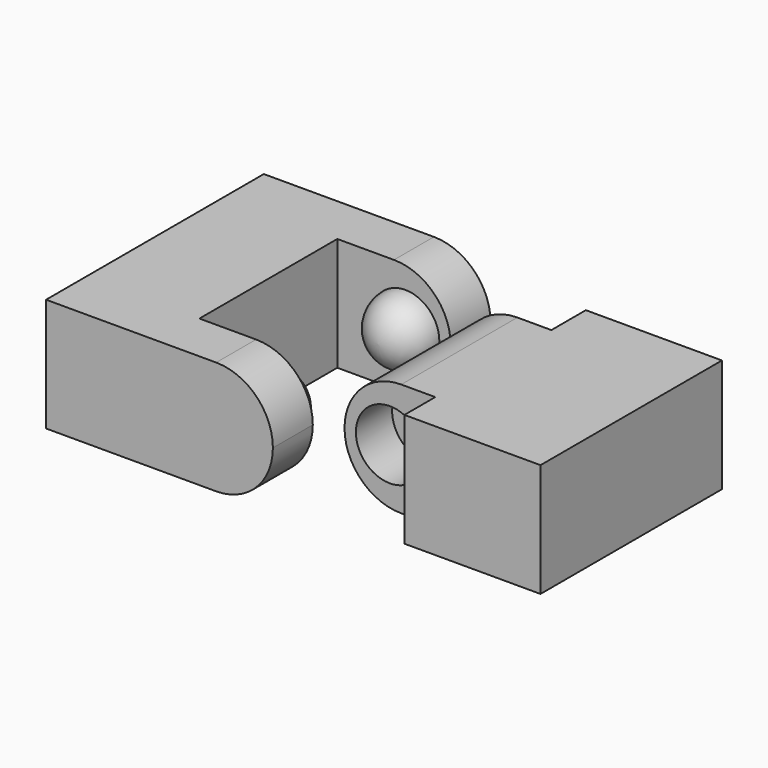
from build123d import *

# Parameters (mm, degrees)
F1_DEPTH  = 5
F2_R      = 1.5
F3_DEPTH  = 1.5
F4_R      = 1.5
F5_DEPTH  = 2
F6_R      = 1.5
F7_DEPTH  = 1.5
F8_R      = 1.49999
F9_W      = 1
F9_H      = 7.6
F10_DEPTH = 5
F11_DEPTH = 1
F12_DEPTH = 1
F13_R     = 2.49999
F13_2_R   = 2.49999
F14_DEPTH = 2
F15_DEPTH = 2
F16_R     = 1.5
F17_DEPTH = 2


# Not quite as in the source:
# - a fillet or chamfer is up to 0.001 mm smaller than in the source, because OpenCascade refuses the exact size


with BuildPart() as f1:
    # F0 (on Top) → F1 (new body)
    with BuildSketch(Plane.XY):
        Polygon((0, 6.4), (0, 0), (4, 0), (4, -1.7), (8, -1.7), (8, 8.3), (4, 8.3), (4, 6.4), align=None)
    extrude(amount=F1_DEPTH)

    # F4 (on face) → F5 (cut)
    with BuildSketch(Plane(origin=(0, 6.4, 0), x_dir=(-1, 0, 0), z_dir=(0, 1, 0))):
        with Locations((-2, 2.5)):
            Circle(F4_R)
    extrude(amount=-F5_DEPTH, mode=Mode.SUBTRACT)

    # F13 (radius 2.5 in the source; OpenCascade refuses exactly that, so slightly less here)
    f13_edges = [f1.edges().sort_by_distance(p)[0] for p in [
        (0, 3.2, 5),
        (0, 3.2, 0),
    ]]
    fillet(f13_edges, radius=F13_R)

    # F14 (add): a face of the model
    f14_faces = [f1.faces().sort_by_distance(p)[0] for p in [
        (8, 3.3, 2.5),
    ]]
    extrude(f14_faces, amount=F14_DEPTH)

    # F16 (on face) → F17 (cut)
    with BuildSketch(Plane.XZ):
        with Locations((2, 2.5)):
            Circle(F16_R)
    extrude(amount=-F17_DEPTH, mode=Mode.SUBTRACT)


with BuildPart() as f1b:
    # F0 (on Top) → F1, piece 2 (new body)
    with BuildSketch(Plane.XY):
        Polygon((-5, 7.1), (-1, 7.1), (-1, 8.3), (-9, 8.3), (-9, -1.7), (-1, -1.7), (-1, -0.5), (-5, -0.5), align=None)
    extrude(amount=F1_DEPTH)

    # F2 (on face) → F3 (join)
    with BuildSketch(Plane.XZ.offset(-7.1)):
        with Locations((-3, 2.5)):
            Circle(F2_R)
    extrude(amount=F3_DEPTH)

    # F6 (on face) → F7 (join)
    with BuildSketch(Plane(origin=(0, -0.5, 0), x_dir=(-1, 0, 0), z_dir=(0, 1, 0))):
        with Locations((3, 2.5)):
            Circle(F6_R)
    extrude(amount=F7_DEPTH)

    # F8 (radius 1.5 in the source; OpenCascade refuses exactly that, so slightly less here)
    f8_edges = [f1b.edges().sort_by_distance(p)[0] for p in [
        (-1.5, 1, 2.5),
        (-4.5, 5.6, 2.5),
    ]]
    fillet(f8_edges, radius=F8_R)

    # F9 (on face) → F10 (cut, through all)
    with BuildSketch(Plane.XY.offset(5)):
        with Locations((-5.5, 3.3)):
            Rectangle(F9_W, F9_H)
    extrude(amount=-F10_DEPTH, mode=Mode.SUBTRACT)

    # F11 (add): a face of the model
    f11_faces = [f1b.faces().sort_by_distance(p)[0] for p in [
        (-5, -1.7, 2.5),
    ]]
    extrude(f11_faces, amount=F11_DEPTH)

    # F12 (add): a face of the model
    f12_faces = [f1b.faces().sort_by_distance(p)[0] for p in [
        (-5, 8.3, 2.5),
    ]]
    extrude(f12_faces, amount=F12_DEPTH)

    # F13#2 (radius 2.5 in the source; OpenCascade refuses exactly that, so slightly less here)
    f13_2_edges = [f1b.edges().sort_by_distance(p)[0] for p in [
        (-1, -1.6, 0),
        (-1, -1.6, 5),
        (-1, 8.2, 5),
        (-1, 8.2, 0),
    ]]
    fillet(f13_2_edges, radius=F13_2_R)

    # F15 (add): a face of the model
    f15_faces = [f1b.faces().sort_by_distance(p)[0] for p in [
        (-9, 3.3, 2.5),
    ]]
    extrude(f15_faces, amount=F15_DEPTH)


solid = Compound([f1.part, f1b.part])
